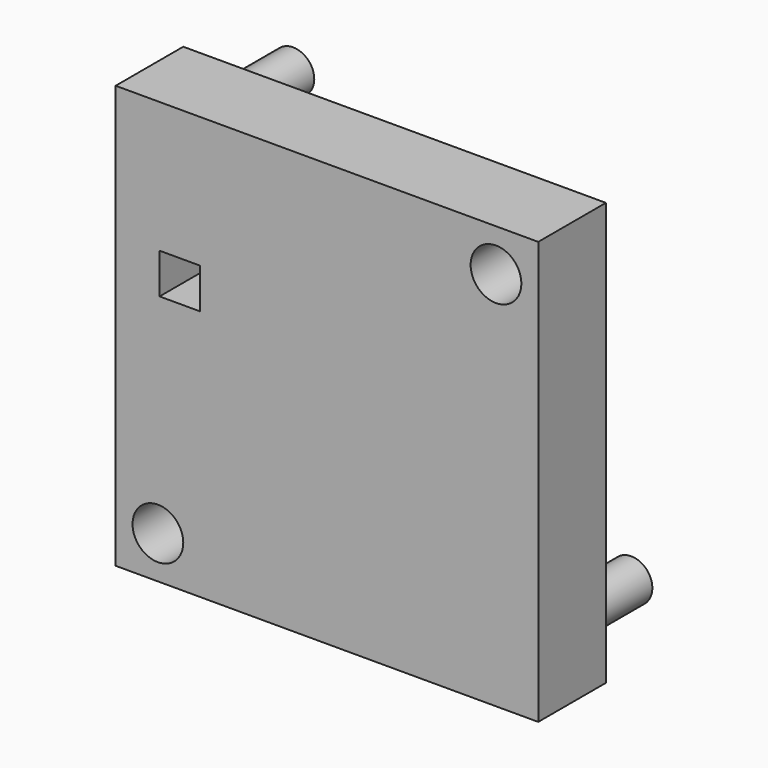
from build123d import *

# Parameters (mm, degrees)
F0_W          = 50
F0_H          = 50
F0_R          = 3
F0_R_2        = 2.5
F1_DEPTH      = 5
F0_W_2        = 4.763
F0_H_2        = 4.763
F2_DEPTH      = 5
F3_DEPTH      = 15
F3_DEPTH_BACK = 5


with BuildPart() as f1:
    # F0 (on Front) → F1 (new body, symmetric)
    with BuildSketch(Plane.XZ):
        with Locations((-17.8228546229, -1.0937498882)):
            Rectangle(F0_W, F0_H)
        with Locations((-37.8228546229, -21.0937498882)):
            Circle(F0_R, mode=Mode.SUBTRACT)
        with Locations((2.1771453771, -21.0937498882)):
            Circle(F0_R_2, mode=Mode.SUBTRACT)
        Polygon((-37.6238546229, 8.4166441185), (-32.8608546229, 8.4166441185), (-16.6755962394, 8.4166441185), (-16.6755962394, 14.7900106385), (-11.9125962394, 14.7900106385), (-11.9125962394, 8.4166441185), (-2.5272074943, 8.4166441185), (-2.5272074943, -12.8520363942), (-13.7815852112, -12.8520363942), (-19.5766687393, -12.8520363942), (-19.5766687393, -10.0679453462), (-27.1787202845, -10.0679453462), (-27.1787202845, -9.4257498882), (-31.0388546229, -9.4257498882), (-31.0388546229, -14.1887498882), (-35.8018546229, -14.1887498882), (-35.8018546229, -9.4257498882), (-35.8018546229, -5.3049453462), (-27.1787202845, -5.3049453462), (-14.8136687393, -5.3049453462), (-14.8136687393, -8.8673923165), (-7.2902074943, -8.8673923165), (-7.2902074943, -4.3980097398), (-14.436878264, -4.3980097398), (-14.436878264, 0.3649902602), (-8.9991306886, 0.3649902602), (-8.9991306886, 3.6536441185), (-16.6755962394, 3.6536441185), (-32.8608546229, 3.6536441185), (-37.6238546229, 3.6536441185), align=None, mode=Mode.SUBTRACT)
        with Locations((-37.8228546229, 18.9062501118)):
            Circle(F0_R_2, mode=Mode.SUBTRACT)
        with Locations((2.1771453771, 18.9062501118)):
            Circle(F0_R, mode=Mode.SUBTRACT)
    extrude(amount=F1_DEPTH, both=True)

    # F0 (on Front) → F2 (join)
    with BuildSketch(Plane.XZ):
        Polygon((-16.6755962394, 8.4166441185), (-32.8608546229, 8.4166441185), (-32.8608546229, 3.6536441185), (-16.6755962394, 3.6536441185), (-8.9991306886, 3.6536441185), (-8.9991306886, 0.3649902602), (-14.436878264, 0.3649902602), (-14.436878264, -4.3980097398), (-7.2902074943, -4.3980097398), (-7.2902074943, -8.8673923165), (-14.8136687393, -8.8673923165), (-14.8136687393, -5.3049453462), (-27.1787202845, -5.3049453462), (-35.8018546229, -5.3049453462), (-35.8018546229, -9.4257498882), (-31.0388546229, -9.4257498882), (-27.1787202845, -9.4257498882), (-27.1787202845, -10.0679453462), (-19.5766687393, -10.0679453462), (-19.5766687393, -12.8520363942), (-13.7815852112, -12.8520363942), (-2.5272074943, -12.8520363942), (-2.5272074943, 8.4166441185), (-11.9125962394, 8.4166441185), (-11.9125962394, 14.7900106385), (-16.6755962394, 14.7900106385), align=None)
        with Locations((-33.4203546229, -11.8072498882)):
            Rectangle(F0_W_2, F0_H_2)
    extrude(amount=F2_DEPTH)

    # F0 (on Front) → F3 (join, two sides)
    with BuildSketch(Plane.XZ) as f3_sk:
        with Locations((2.1771453771, -21.0937498882)):
            Circle(F0_R_2)
        with Locations((-37.8228546229, 18.9062501118)):
            Circle(F0_R_2)
    extrude(amount=-F3_DEPTH)
    extrude(f3_sk.sketch, amount=F3_DEPTH_BACK)


solid = f1.part
